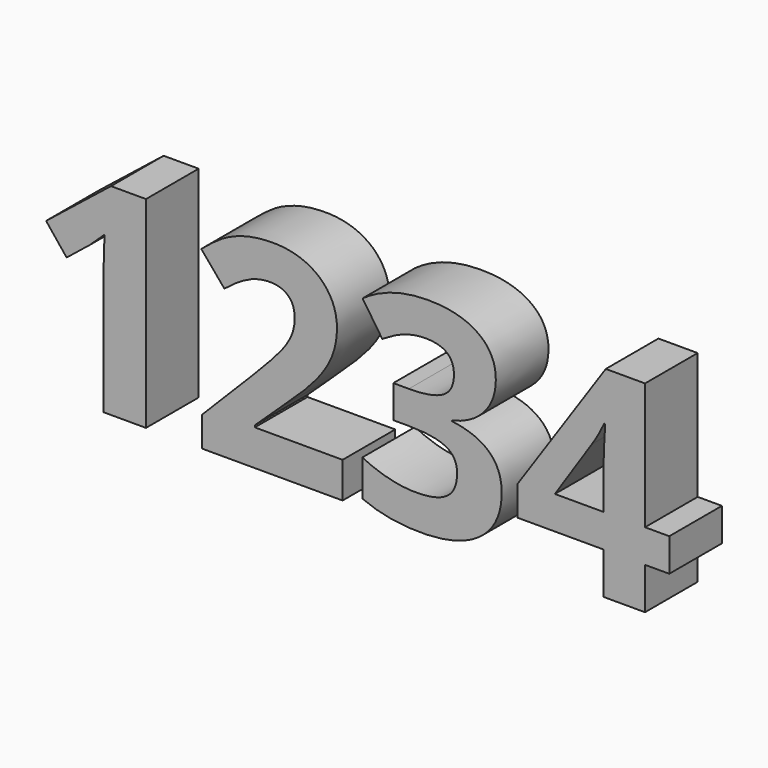
from build123d import *

# Parameters (mm, degrees)
F1_TEXT_SIZE = 51.4503919073
F3_DEPTH     = 12


# Not quite as in the source:
# - a feature of the source that left no trace in its solid (it failed there, or was rolled back) is left out
# - Text() gives the source's letters only with a copy of the font that has no kerning and outlines rounded to 1/6400 em; it was checked with that copy


with BuildPart() as f3:
    # F1 (on face) → F3 (new body)
    with BuildSketch(Plane.XZ):
        with Locations((0, -37.0442821732)):
            Text('1234', F1_TEXT_SIZE, font='Open Sans', font_style=FontStyle.BOLD, text_align=(TextAlign.LEFT, TextAlign.BOTTOM))
    extrude(amount=-F3_DEPTH)


with BuildPart() as f3_1:
    # F4: moved
    add(f3.part.moved(Location((0, 0, 25))))


solid = f3_1.part
